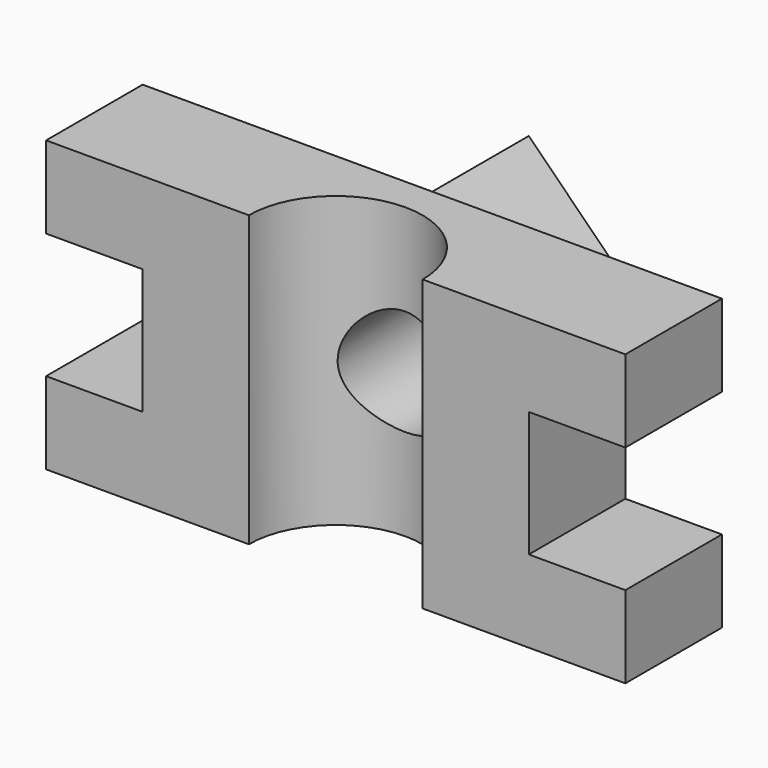
from build123d import *

# Parameters (mm, degrees)
F1_DEPTH = 250
F3_DEPTH = 600.001
F5_DEPTH = 250
F6_R     = 110
F7_DEPTH = 500.001


# Not quite as in the source:
# - a feature names something its author has since deleted; it is built from what else it names


with BuildPart() as f1:
    # F0 (on Front) → F1 (new body)
    with BuildSketch(Plane.XZ):
        Polygon((-600, -300), (600, -300), (600, -130), (400, -130), (400, 130), (600, 130), (600, 300), (-600, 300), (-600, 130), (-400, 130), (-400, -130), (-600, -130), align=None)
    extrude(amount=F1_DEPTH)

    # F2 (on face) → F3 (cut, through all)
    with BuildSketch(Plane.XY.offset(300)):
        with BuildLine():
            Line((-180, -250), (180, -250))
            ThreePointArc((180, -250), (0, -70), (-180, -250))
        make_face()
    extrude(amount=-F3_DEPTH, mode=Mode.SUBTRACT)

    # F4 (on face) → F5 (join)
    with BuildSketch(Plane(origin=(0, 0, 0), x_dir=(-1, 0, 0), z_dir=(0, 1, 0))):
        Polygon((0, 300), (-300, 0), (0, -300), (300, 0), align=None)
    extrude(amount=F5_DEPTH)

    # F6 (on face) → F7 (cut, through all)
    with BuildSketch(Plane(origin=(0, 250, 0), x_dir=(-1, 0, 0), z_dir=(0, 1, 0))):
        Circle(F6_R)
    extrude(amount=-F7_DEPTH, mode=Mode.SUBTRACT)


solid = f1.part
